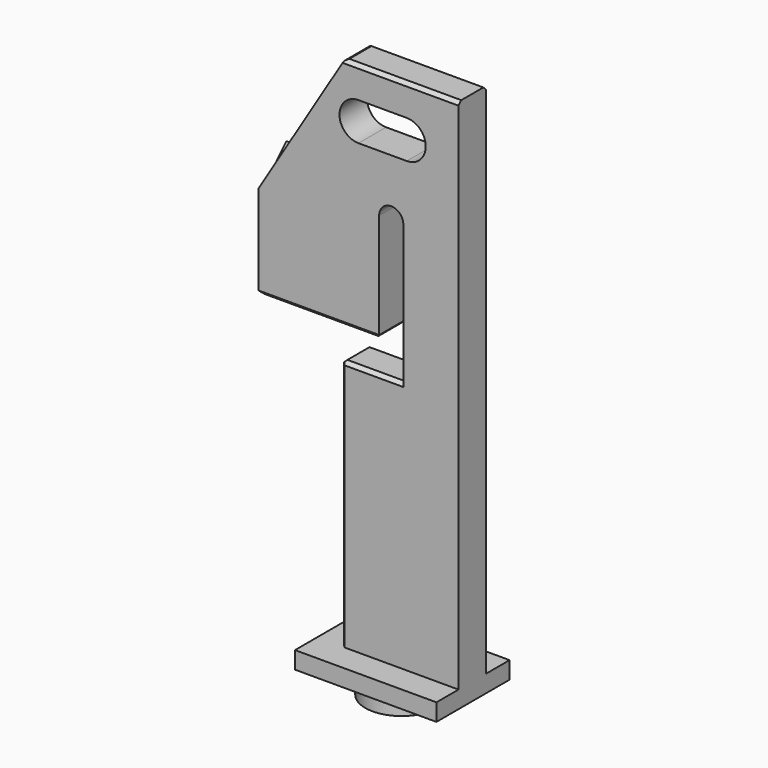
from build123d import *

# Parameters (mm, degrees)
F1_DEPTH     = 20
F2_W         = 14
F2_H         = 63
F3_DEPTH     = 25
F4_W         = 28
F4_H         = 22
F5_DEPTH     = 25
F7_DEPTH     = 16
F10_DEPTH    = 17
F9_R         = 21
F11_DEPTH    = 10
F13_SIZE     = 2
F14_T1_DEPTH = 30.2867319519
F14_T3_DEPTH = 26.2867319519
F14_T5_DEPTH = 25.9668324626
F15_SIZE     = 2
F18_W        = 68.8039958477
F18_H        = 47.8929802775
F19_DEPTH    = 10


# Not quite as in the source:
# - a fillet or chamfer that OpenCascade refuses, or shapes differently, is made with other operations: its cross-section is extruded or revolved along the edge and cut away or added


with BuildPart() as f1:
    # F0 (on Front) → F1 (new body)
    with BuildSketch(Plane.XZ):
        Polygon((-30.5923320651, 260.9896056354), (-146.5923320651, 260.9896056354), (-146.5923320651, -39.0103943646), (-112.5923320651, -39.0103943646), (-30.5923320651, -39.0103943646), align=None)
        Polygon((-30.5923320651, -49.0103943646), (-30.5923320651, -39.0103943646), (-112.5923320651, -39.0103943646), (-112.5923320651, -49.0103943646), (-92.5923320651, -49.0103943646), (-50.5923320651, -49.0103943646), align=None)
    extrude(amount=-F1_DEPTH)

    # F2 (on face) → F3 (cut)
    with BuildSketch(Plane.XZ):
        Polygon((-158.5923320651, 124.9896056354), (-158.5923320651, -39.0103943646), (-98.5923320651, -39.0103943646), (-98.5923320651, 106.9896056354), (-98.5923320651, 124.9896056354), align=None)
        Polygon((-98.5923320651, 124.9896056354), (-98.5923320651, 106.9896056354), (-62.5923320651, 106.9896056354), (-62.5923320651, 124.9896056354), (-76.5923320651, 124.9896056354), align=None)
        with Locations((-69.5923320651, 156.4896056354)):
            Rectangle(F2_W, F2_H)
        with BuildLine():
            ThreePointArc((-62.5923320651, 187.9896056354), (-69.5923320651, 194.9896056354), (-76.5923320651, 187.9896056354))
            Line((-76.5923320651, 187.9896056354), (-62.5923320651, 187.9896056354))
        make_face()
        Polygon((-146.5923320651, 260.9896056354), (-146.5923320651, 178.9896056354), (-96.5923320651, 260.9896056354), align=None)
    extrude(amount=-F3_DEPTH, mode=Mode.SUBTRACT)

    # F4 (on face) → F5 (cut)
    with BuildSketch(Plane.XZ):
        with Locations((-74.5923320651, 231.9896056354)):
            Rectangle(F4_W, F4_H)
        with BuildLine():
            ThreePointArc((-60.5923320651, 220.9896056354), (-49.5923320651, 231.9896056354), (-60.5923320651, 242.9896056354))
            Line((-60.5923320651, 242.9896056354), (-60.5923320651, 220.9896056354))
        make_face()
        with BuildLine():
            Line((-88.5923320651, 220.9896056354), (-88.5923320651, 242.9896056354))
            ThreePointArc((-88.5923320651, 242.9896056354), (-99.5923320651, 231.9896056354), (-88.5923320651, 220.9896056354))
        make_face()
    extrude(amount=-F5_DEPTH, mode=Mode.SUBTRACT)

    # F6 (on face) → F7 (join)
    with BuildSketch(Plane.XZ):
        Polygon((-30.5923320651, -39.0103943646), (-98.5923320651, -39.0103943646), (-112.5923320651, -39.0103943646), (-112.5923320651, -49.0103943646), (-30.5923320651, -49.0103943646), align=None)
    extrude(amount=F7_DEPTH)

    # F8 (on face) → F10 (join)
    with BuildSketch(Plane(origin=(0, 20, 0), x_dir=(-1, 0, 0), z_dir=(0, 1, 0))):
        Polygon((112.5923320651, -39.0103943646), (98.5923320651, -39.0103943646), (30.5923320651, -39.0103943646), (30.5923320651, -49.0103943646), (112.5923320651, -49.0103943646), align=None)
    extrude(amount=F10_DEPTH)

    # F9 (on face) → F11 (join)
    with BuildSketch(Plane(origin=(0, 0, -49.0103943646), x_dir=(1, 0, 0), z_dir=(0, 0, -1))):
        with Locations((-71.5923320651, -10)):
            Circle(F9_R)
    extrude(amount=F11_DEPTH)

    # F13
    f13_edges = [f1.edges().sort_by_distance(p)[0] for p in [
        (-98.592332, 0, 33.989606),
        (-98.592332, 20, 33.989606),
    ]]
    chamfer(f13_edges, length=F13_SIZE)

    # F14: chamfer of 2 on 4 edges, made by hand

    # F14_s2 → F14_t1 (cut)
    with BuildSketch(Plane.XZ.offset(-25.1433659759)):
        Polygon((-146.5923320651, 126.9896056354), (-144.5923320651, 124.9896056354), (-146.5923320651, 124.9896056354), align=None)
        Polygon((-76.5923320651, 126.9896056354), (-78.5923320651, 124.9896056354), (-76.5923320651, 124.9896056354), align=None)
    extrude(amount=F14_T1_DEPTH, mode=Mode.SUBTRACT)

    # F14_s4 → F14_t3 (cut)
    with BuildSketch(Plane.XZ.offset(-23.1433659759)):
        Polygon((-96.5923320651, 106.9896056354), (-98.5923320651, 104.9896056354), (-98.5923320651, 106.9896056354), align=None)
    extrude(amount=F14_T3_DEPTH, mode=Mode.SUBTRACT)

    # F14_s6 → F14_t5 (cut)
    with BuildSketch(Plane.XZ.offset(-22.9834162313)):
        Polygon((-95.4693648059, 260.9896056354), (-97.1769571575, 260.0308204839), (-96.5923320651, 260.9896056354), align=None)
    extrude(amount=F14_T5_DEPTH, mode=Mode.SUBTRACT)

    # F15
    f15_edges = [f1.edges().sort_by_distance(p)[0] for p in [
        (-111.592332, 0, 124.989606),
        (-111.592332, 20, 124.989606),
        (-79.592332, 0, 106.989606),
        (-79.592332, 20, 106.989606),
        (-63.030848, 0, 260.989606),
        (-63.030848, 20, 260.989606),
    ]]
    chamfer(f15_edges, length=F15_SIZE)

    # F18 (on face) → F19 (join)
    with BuildSketch(Plane(origin=(0, 107.4948028177, 107.4948028177), x_dir=(1, 0, 0), z_dir=(0, -0.7071067812, -0.7071067812))):
        with Locations((-111.8147820234, 100.1271270216)):
            Rectangle(F18_W, F18_H)
    extrude(amount=F19_DEPTH)


solid = f1.part
